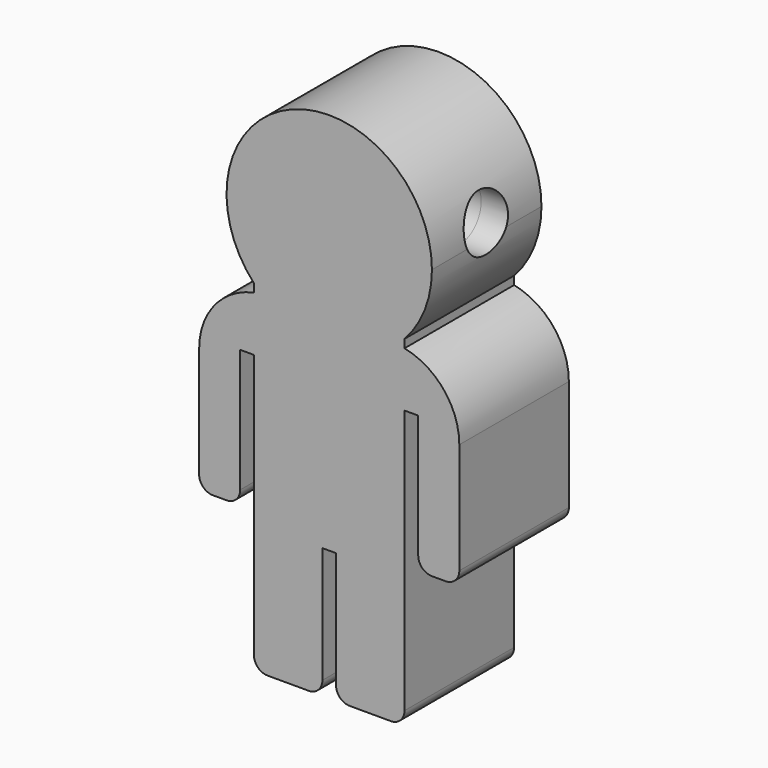
from build123d import *

# Parameters (mm, degrees)
F1_DEPTH      = 10
F2_T1_DEPTH   = 34.4948974279
F3_R          = 1
F4_SCALE      = 0.5
F5_R          = 1
F6_DEPTH      = 25
F6_DEPTH_BACK = 25


# Not quite as in the source:
# - a fillet or chamfer that OpenCascade refuses, or shapes differently, is made with other operations: its cross-section is extruded or revolved along the edge and cut away or added


with BuildPart() as f1:
    # F0 (on Front) → F1 (new body)
    with BuildSketch(Plane.XZ):
        with BuildLine():
            Line((-11, 11.2686367076), (-11, 16.3676562212))
            Line((-11, 16.3676562212), (0, 16.3676562212))
            Line((0, 16.3676562212), (0, 11.2686367076))
            ThreePointArc((0, 11.2686367076), (1.4821200219, 13.6290434337), (2, 16.3676562212))
            ThreePointArc((2, 16.3676562212), (-8.2386127875, 23.3497762431), (-11, 11.2686367076))
        make_face()
        with BuildLine():
            Line((0, 16.3676562212), (-11, 16.3676562212))
            Line((-11, 16.3676562212), (-11, 11.2686367076))
            ThreePointArc((-11, 11.2686367076), (-5.5, 8.8676562212), (0, 11.2686367076))
            Line((0, 11.2686367076), (0, 16.3676562212))
        make_face()
        with BuildLine():
            ThreePointArc((0, 11.2686367076), (-5.5, 8.8676562212), (-11, 11.2686367076))
            Line((-11, 11.2686367076), (-11, 10.6633629519))
            Line((-11, 10.6633629519), (-11, 6.6633629519))
            Line((-11, 6.6633629519), (-11, -3.3366370481))
            Line((-11, -3.3366370481), (-11, -13.6323437788))
            Line((-11, -13.6323437788), (-6, -13.6323437788))
            Line((-6, -13.6323437788), (-6, -4.1323437788))
            Line((-6, -4.1323437788), (-5, -4.1323437788))
            Line((-5, -4.1323437788), (-5, -13.6323437788))
            Line((-5, -13.6323437788), (0, -13.6323437788))
            Line((0, -13.6323437788), (0, -3.3363437788))
            Line((0, -3.3363437788), (0, 6.6636562212))
            Line((0, 6.6636562212), (0, 10.6636562212))
            Line((0, 10.6636562212), (0, 11.2686367076))
        make_face()
        Polygon((-11, 6.6633629519), (-11, 10.6633629519), (-15, 10.6633629519), (-15, -3.3366370481), (-12, -3.3366370481), (-12, 6.6633629519), align=None)
        Polygon((4, 10.6636562212), (0, 10.6636562212), (0, 6.6636562212), (1, 6.6636562212), (1, -3.3363437788), (4, -3.3363437788), align=None)
    extrude(amount=F1_DEPTH)

    # F2: fillet of radius 5 on 2 edges, made by hand

    # F2_s2 → F2_t1 (cut)
    with BuildSketch(Plane.XZ.offset(-12.2474487139)):
        with BuildLine():
            ThreePointArc((4, 5.7646767356), (2.8729833462, 8.9269543958), (0, 10.6636562212))
            Line((0, 10.6636562212), (4, 10.6636562212))
            Line((4, 10.6636562212), (4, 5.7646767356))
        make_face()
        with BuildLine():
            ThreePointArc((-11, 10.6633629519), (-13.8729833462, 8.9266611265), (-15, 5.7643834664))
            Line((-15, 5.7643834664), (-15, 10.6633629519))
            Line((-15, 10.6633629519), (-11, 10.6633629519))
        make_face()
    extrude(amount=F2_T1_DEPTH, mode=Mode.SUBTRACT)

    # F3
    f3_edges = [f1.edges().sort_by_distance(p)[0] for p in [
        (-15, -5, -3.336637),
        (-12, -5, -3.336637),
        (1, -5, -3.336344),
        (4, -5, -3.336344),
        (-5, -5, -13.632344),
        (0, -5, -13.632344),
        (-11, -5, -13.632344),
        (-6, -5, -13.632344),
    ]]
    fillet(f3_edges, radius=F3_R)


with BuildPart() as f1_1:
    # F4: moved
    add(f1.part.scale(F4_SCALE))

    # F5 (on Right) → F6 (cut, two sides)
    with BuildSketch(Plane.YZ) as f6_sk:
        with Locations((-2.5, 8.6343183538)):
            Circle(F5_R)
    extrude(amount=-F6_DEPTH, mode=Mode.SUBTRACT)
    extrude(f6_sk.sketch, amount=F6_DEPTH_BACK, mode=Mode.SUBTRACT)


solid = f1_1.part
